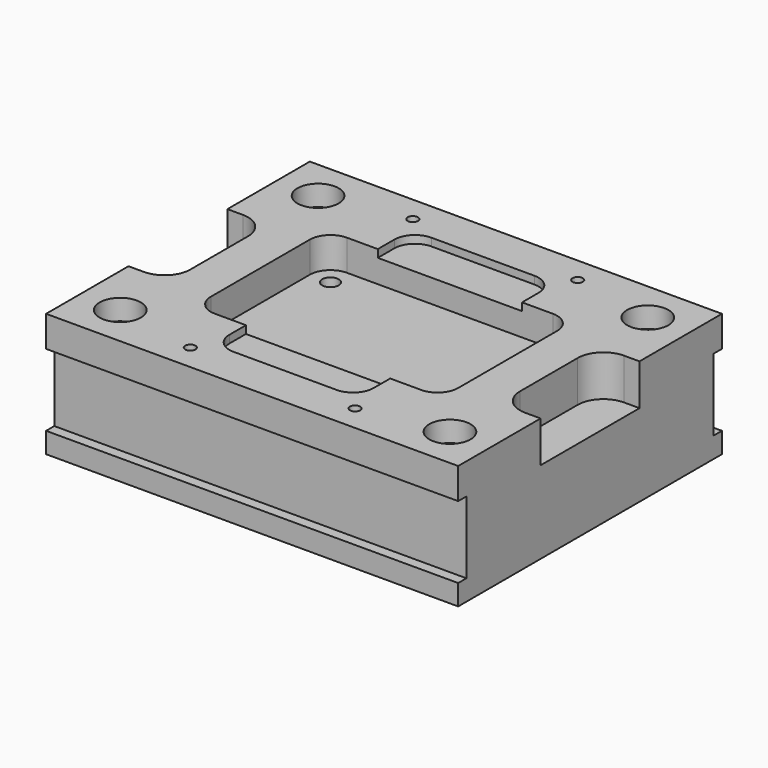
from build123d import *

# Parameters (mm, degrees)
F0_W           = 127
F0_H           = 101.6
F1_DEPTH       = 38.1
F2_W           = 76.2
F2_H           = 50.8
F3_DEPTH       = 9.525
F4_R           = 6.35
F6_D           = 6.35
F6_CBORE_D     = 12.7
F6_CBORE_DEPTH = 6.35
F7_W           = 3.175
F7_H           = 22.225
F8_DEPTH       = 127.001
F10_D          = 5.1054
F10_DEPTH      = 19.05
F10_TIP        = 1.5338169022
F11_W          = 12.7
F11_H          = 38.1
F12_DEPTH      = 12.7
F13_R          = 7.9375
F15_DEPTH      = 3.175
F16_W          = 57.15
F16_H          = 31.75
F17_DEPTH      = 6.35
F18_R          = 6.35
F20_D          = 3.175
F20_DEPTH      = 9.525
F20_TIP        = 0.9538662327
F21_W          = 44.45
F21_H          = 76.2
F22_DEPTH      = 2.38125
F23_R          = 6.35


# Not quite as in the source:
# - a feature of the source that left no trace in its solid (it failed there, or was rolled back) is left out


with BuildPart() as f1:
    # F0 (on Top) → F1 (new body)
    with BuildSketch(Plane.XY):
        Rectangle(F0_W, F0_H)
    extrude(amount=F1_DEPTH)

    # F2 (on face) → F3 (cut)
    with BuildSketch(Plane.XY.offset(38.1)):
        Rectangle(F2_W, F2_H)
    extrude(amount=-F3_DEPTH, mode=Mode.SUBTRACT)

    # F4
    f4_edges = [f1.edges().sort_by_distance(p)[0] for p in [
        (-38.1, 25.4, 33.3375),
        (38.1, 25.4, 33.3375),
        (38.1, -25.4, 33.3375),
        (-38.1, -25.4, 33.3375),
    ]]
    fillet(f4_edges, radius=F4_R)

    # F6 (through all)
    with Locations(Plane.XY.offset(38.1)):
        with Locations((-50.8, 38.1), (50.8, 38.1), (50.8, -38.1), (-50.8, -38.1)):
            CounterBoreHole(F6_D / 2, F6_CBORE_D / 2, F6_CBORE_DEPTH)

    # F7 (on face) → F8 (cut, through all)
    with BuildSketch(Plane.YZ.offset(63.5)):
        with Locations((-49.2125, 17.4625)):
            Rectangle(F7_W, F7_H)
        with Locations((49.2125, 17.4625)):
            Rectangle(F7_W, F7_H)
    extrude(amount=-F8_DEPTH, mode=Mode.SUBTRACT)

    # F10
    with Locations(Plane.XY.offset(28.575)):
        with Locations((-31.75, 19.05), (-31.75, -19.05), (31.75, -19.05), (31.75, 19.05)):
            Hole(F10_D / 2, depth=F10_DEPTH)
            with Locations((0, 0, -(F10_DEPTH + F10_TIP / 2))):  # 118° drill point
                Cone(0, F10_D / 2, F10_TIP, mode=Mode.SUBTRACT)

    # F11 (on face) → F12 (cut)
    with BuildSketch(Plane.XY.offset(38.1)):
        with Locations((-57.15, 0)):
            Rectangle(F11_W, F11_H)
        with Locations((57.15, 0)):
            Rectangle(F11_W, F11_H)
    extrude(amount=-F12_DEPTH, mode=Mode.SUBTRACT)

    # F13
    f13_edges = [f1.edges().sort_by_distance(p)[0] for p in [
        (-50.8, 19.05, 31.75),
        (-50.8, -19.05, 31.75),
        (50.8, 19.05, 31.75),
        (50.8, -19.05, 31.75),
    ]]
    fillet(f13_edges, radius=F13_R)

    # F14 (on face) → F15 (cut)
    with BuildSketch(Plane(origin=(0, 0, 0), x_dir=(1, 0, 0), z_dir=(0, 0, -1))):
        with BuildLine():
            Line((-31.75, -25.4), (31.75, -25.4))
            ThreePointArc((31.75, -25.4), (36.2401280605, -23.5401280605), (38.1, -19.05))
            Line((38.1, -19.05), (38.1, 19.05))
            ThreePointArc((38.1, 19.05), (36.2401280605, 23.5401280605), (31.75, 25.4))
            Line((31.75, 25.4), (-31.75, 25.4))
            ThreePointArc((-31.75, 25.4), (-36.2401280605, 23.5401280605), (-38.1, 19.05))
            Line((-38.1, 19.05), (-38.1, -19.05))
            ThreePointArc((-38.1, -19.05), (-36.2401280605, -23.5401280605), (-31.75, -25.4))
        make_face()
    extrude(amount=-F15_DEPTH, mode=Mode.SUBTRACT)

    # F16 (on face) → F17 (cut)
    with BuildSketch(Plane(origin=(0, 0, 3.175), x_dir=(1, 0, 0), z_dir=(0, 0, -1))):
        Rectangle(F16_W, F16_H)
    extrude(amount=-F17_DEPTH, mode=Mode.SUBTRACT)

    # F18
    f18_edges = [f1.edges().sort_by_distance(p)[0] for p in [
        (-28.575, -15.875, 6.35),
        (-28.575, 15.875, 6.35),
        (28.575, -15.875, 6.35),
        (28.575, 15.875, 6.35),
    ]]
    fillet(f18_edges, radius=F18_R)

    # F20
    with Locations(Plane.XY.offset(38.1)):
        with Locations((-25.4, 42.8625), (25.4, 42.8625), (-25.4, -42.8625), (25.4, -42.8625)):
            Hole(F20_D / 2, depth=F20_DEPTH)
            with Locations((0, 0, -(F20_DEPTH + F20_TIP / 2))):  # 118° drill point
                Cone(0, F20_D / 2, F20_TIP, mode=Mode.SUBTRACT)

    # F21 (on face) → F22 (cut)
    with BuildSketch(Plane.XY.offset(38.1)):
        Rectangle(F21_W, F21_H)
    extrude(amount=-F22_DEPTH, mode=Mode.SUBTRACT)

    # F23
    f23_edges = [f1.edges().sort_by_distance(p)[0] for p in [
        (-22.225, 38.1, 36.909375),
        (22.225, 38.1, 36.909375),
        (22.225, -38.1, 36.909375),
        (-22.225, -38.1, 36.909375),
    ]]
    fillet(f23_edges, radius=F23_R)


solid = f1.part
